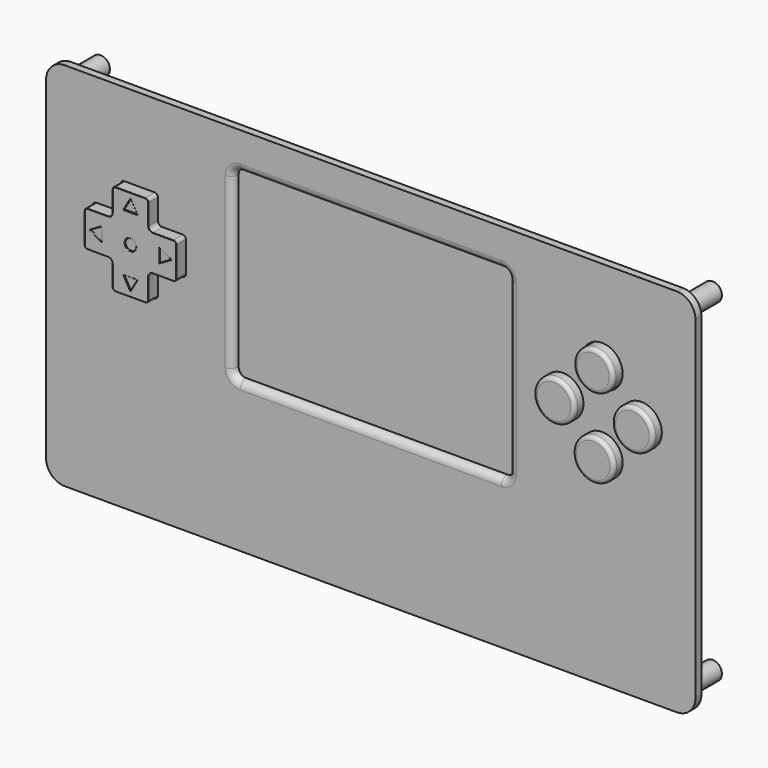
from build123d import *

# Parameters (mm, degrees)
F0_W           = 174
F0_H           = 99.3
F0_R           = 17.5
F0_W_2         = 74
F0_H_2         = 49.3
F0_R_2         = 5.5
F1_DEPTH       = 2
F2_R           = 1
F3_R           = 5
F4_R           = 6.5
F4_R_2         = 5.5
F5_DEPTH       = 5
F6_R           = 19.5
F6_R_2         = 17.5
F7_DEPTH       = 5
F8_R           = 1.99999
F9_R           = 2.5
F9_R_2         = 1
F10_DEPTH      = 10
F11_DEPTH      = 2
F13_DEPTH      = 3
F13_DEPTH_BACK = 3
F14_R          = 5.3
F15_DEPTH      = 3
F15_DEPTH_BACK = 2
F14_R_2        = 5.5
F16_R          = 1
F16_2_R        = 1
F16_3_R        = 1
F16_4_R        = 1
F17_R          = 1.5
F18_DEPTH      = 0.2
F19_R          = 0.09999


# Not quite as in the source:
# - a fillet or chamfer is up to 0.001 mm smaller than in the source, because OpenCascade refuses the exact size


with BuildPart() as f1:
    # F0 (on Front) → F1 (new body)
    with BuildSketch(Plane.XZ):
        with Locations((0, -15)):
            Rectangle(F0_W, F0_H)
        with Locations((-62, 0)):
            Circle(F0_R, mode=Mode.SUBTRACT)
        Rectangle(F0_W_2, F0_H_2, mode=Mode.SUBTRACT)
        with Locations((62, -10.5)):
            Circle(F0_R_2, mode=Mode.SUBTRACT)
        with Locations((51.5, 0)):
            Circle(F0_R_2, mode=Mode.SUBTRACT)
        with Locations((72.5, 0)):
            Circle(F0_R_2, mode=Mode.SUBTRACT)
        with Locations((62, 10.5)):
            Circle(F0_R_2, mode=Mode.SUBTRACT)
        with Locations((-62, 0)):
            Circle(F0_R)
        Polygon((-57, -5), (-57, -12.5), (-67, -12.5), (-67, -5), (-74.5, -5), (-74.5, 5), (-67, 5), (-67, 12.5), (-57, 12.5), (-57, 5), (-49.5, 5), (-49.5, -5), align=None, mode=Mode.SUBTRACT)
    extrude(amount=F1_DEPTH)

    # F2
    f2_edges = [f1.edges().sort_by_distance(p)[0] for p in [
        (-67, -1, 12.5),
        (-67, -1, 5),
        (-74.5, -1, 5),
        (-74.5, -1, -5),
        (-67, -1, -5),
        (-67, -1, -12.5),
        (-57, -1, -12.5),
        (-57, -1, -5),
        (-49.5, -1, -5),
        (-49.5, -1, 5),
        (-57, -1, 5),
        (-57, -1, 12.5),
    ]]
    fillet(f2_edges, radius=F2_R)

    # F3
    f3_edges = [f1.edges().sort_by_distance(p)[0] for p in [
        (87, -1, 34.65),
        (87, -1, -64.65),
        (-87, -1, 34.65),
        (-87, -1, -64.65),
    ]]
    fillet(f3_edges, radius=F3_R)

    # F4 (on face) → F5 (join)
    with BuildSketch(Plane(origin=(0, 0, 0), x_dir=(-1, 0, 0), z_dir=(0, 1, 0))):
        with Locations((-62, 10.5)):
            Circle(F4_R)
        with Locations((-62, 10.5)):
            Circle(F4_R_2, mode=Mode.SUBTRACT)
        with Locations((-72.5, 0)):
            Circle(F4_R)
        with Locations((-72.5, 0)):
            Circle(F4_R_2, mode=Mode.SUBTRACT)
        with Locations((-51.5, 0)):
            Circle(F4_R)
        with Locations((-51.5, 0)):
            Circle(F4_R_2, mode=Mode.SUBTRACT)
        with Locations((-62, -10.5)):
            Circle(F4_R)
        with Locations((-62, -10.5)):
            Circle(F4_R_2, mode=Mode.SUBTRACT)
    extrude(amount=F5_DEPTH)

    # F6 (on face) → F7 (join, through all)
    with BuildSketch(Plane.XZ):
        with Locations((-62, 0)):
            Circle(F6_R)
        with Locations((-62, 0)):
            Circle(F6_R_2, mode=Mode.SUBTRACT)
    extrude(amount=-F7_DEPTH)

    # F8 (radius 2 in the source; OpenCascade refuses exactly that, so slightly less here)
    f8_edges = [f1.edges().sort_by_distance(p)[0] for p in [
        (-37, -1, 24.65),
        (37, -1, 24.65),
        (37, -1, -24.65),
        (-37, -1, -24.65),
        (-37, -2, 0),
        (37, -2, 0),
        (0, -2, 24.65),
        (0, -2, -24.65),
    ]]
    fillet(f8_edges, radius=F8_R)

    # F9 (on face) → F10 (join)
    with BuildSketch(Plane.XZ):
        with Locations((82, 29.65)):
            Circle(F9_R)
        with Locations((82, 29.65)):
            Circle(F9_R_2, mode=Mode.SUBTRACT)
        with Locations((-82, 29.65)):
            Circle(F9_R)
        with Locations((-82, 29.65)):
            Circle(F9_R_2, mode=Mode.SUBTRACT)
        with Locations((-82, -59.65)):
            Circle(F9_R)
        with Locations((-82, -59.65)):
            Circle(F9_R_2, mode=Mode.SUBTRACT)
        with Locations((82, -59.65)):
            Circle(F9_R)
        with Locations((82, -59.65)):
            Circle(F9_R_2, mode=Mode.SUBTRACT)
    extrude(amount=-F10_DEPTH)


with BuildPart() as f11:
    # F0 (on Front) → F11 (new body)
    with BuildSketch(Plane.XZ):
        Rectangle(F0_W_2, F0_H_2)
    extrude(amount=-F11_DEPTH)


with BuildPart() as f13:
    # F12 (on face) → F13 (new body, two sides)
    with BuildSketch(Plane.XZ.offset(2)) as f13_sk:
        with BuildLine():
            ThreePointArc((-66.8, 6), (-67.1514718626, 5.1514718626), (-68, 4.8))
            Line((-68, 4.8), (-73.5, 4.8))
            ThreePointArc((-73.5, 4.8), (-74.0656854249, 4.5656854249), (-74.3, 4))
            Line((-74.3, 4), (-74.3, -4))
            ThreePointArc((-74.3, -4), (-74.0656854249, -4.5656854249), (-73.5, -4.8))
            Line((-73.5, -4.8), (-68, -4.8))
            ThreePointArc((-68, -4.8), (-67.1514718626, -5.1514718626), (-66.8, -6))
            Line((-66.8, -6), (-66.8, -11.5))
            ThreePointArc((-66.8, -11.5), (-66.5656854249, -12.0656854249), (-66, -12.3))
            Line((-66, -12.3), (-58, -12.3))
            ThreePointArc((-58, -12.3), (-57.4343145751, -12.0656854249), (-57.2, -11.5))
            Line((-57.2, -11.5), (-57.2, -6))
            ThreePointArc((-57.2, -6), (-56.8485281374, -5.1514718626), (-56, -4.8))
            Line((-56, -4.8), (-50.5, -4.8))
            ThreePointArc((-50.5, -4.8), (-49.9343145751, -4.5656854249), (-49.7, -4))
            Line((-49.7, -4), (-49.7, 4))
            ThreePointArc((-49.7, 4), (-49.9343145751, 4.5656854249), (-50.5, 4.8))
            Line((-50.5, 4.8), (-56, 4.8))
            ThreePointArc((-56, 4.8), (-56.8485281374, 5.1514718626), (-57.2, 6))
            Line((-57.2, 6), (-57.2, 11.5))
            ThreePointArc((-57.2, 11.5), (-57.4343145751, 12.0656854249), (-58, 12.3))
            Line((-58, 12.3), (-66, 12.3))
            ThreePointArc((-66, 12.3), (-66.5656854249, 12.0656854249), (-66.8, 11.5))
            Line((-66.8, 11.5), (-66.8, 6))
        make_face()
    extrude(amount=F13_DEPTH)
    extrude(f13_sk.sketch, amount=-F13_DEPTH_BACK)

    # F17 (on face) → F18 (cut)
    with BuildSketch(Plane.XZ.offset(5)):
        Polygon((-62, 10.8974880576), (-63.8597792122, 7.6762559712), (-60.1402207878, 7.6762559712), align=None)
        Polygon((-54.3237440288, 1.8597792122), (-54.3237440288, -1.8597792122), (-51.1025119424, 0), align=None)
        Polygon((-62, -10.8974880576), (-60.1402207878, -7.6762559712), (-63.8597792122, -7.6762559712), align=None)
        Polygon((-72.8974880576, 0), (-69.6762559712, -1.8597792122), (-69.6762559712, 1.8597792122), align=None)
        with Locations((-62, 0)):
            Circle(F17_R)
    extrude(amount=-F18_DEPTH, mode=Mode.SUBTRACT)

    # F19 (radius 0.1 in the source; OpenCascade refuses exactly that, so slightly less here)
    f19_edges = [f13.edges().sort_by_distance(p)[0] for p in [
        (-63.5, -4.8, 0),
        (-70.75, -5, -4.8),
        (-74.065685, -5, -4.565685),
        (-67.151472, -5, -5.151472),
        (-74.3, -5, 0),
        (-66.8, -5, -8.75),
        (-74.065685, -5, 4.565685),
        (-66.565685, -5, -12.065685),
        (-70.75, -5, 4.8),
        (-62, -5, -12.3),
        (-67.151472, -5, 5.151472),
        (-57.434315, -5, -12.065685),
        (-66.8, -5, 8.75),
        (-57.2, -5, -8.75),
        (-66.565685, -5, 12.065685),
        (-56.848528, -5, -5.151472),
        (-62, -5, 12.3),
        (-53.25, -5, -4.8),
        (-57.434315, -5, 12.065685),
        (-49.934315, -5, -4.565685),
        (-57.2, -5, 8.75),
        (-49.7, -5, 0),
        (-56.848528, -5, 5.151472),
        (-49.934315, -5, 4.565685),
        (-53.25, -5, 4.8),
        (-71.286872, -5, -0.92989),
        (-69.676256, -5, 0),
        (-71.286872, -5, 0.92989),
        (-62.92989, -5, -9.286872),
        (-61.07011, -5, -9.286872),
        (-62, -5, -7.676256),
        (-63.5, -5, 0),
        (-54.323744, -5, 0),
        (-52.713128, -5, -0.92989),
        (-52.713128, -5, 0.92989),
        (-62.92989, -5, 9.286872),
        (-62, -5, 7.676256),
        (-61.07011, -5, 9.286872),
        (-63.859779, -4.9, 7.676256),
        (-62, -4.9, 10.897488),
        (-62, -4.8, 7.676256),
        (-61.07011, -4.8, 9.286872),
        (-62.92989, -4.8, 9.286872),
        (-60.140221, -4.9, 7.676256),
        (-54.323744, -4.8, 0),
        (-52.713128, -4.8, -0.92989),
        (-52.713128, -4.8, 0.92989),
        (-54.323744, -4.9, -1.859779),
        (-51.102512, -4.9, 0),
        (-54.323744, -4.9, 1.859779),
        (-63.859779, -4.9, -7.676256),
        (-60.140221, -4.9, -7.676256),
        (-62, -4.9, -10.897488),
        (-62.92989, -4.8, -9.286872),
        (-61.07011, -4.8, -9.286872),
        (-62, -4.8, -7.676256),
        (-71.286872, -4.8, -0.92989),
        (-71.286872, -4.8, 0.92989),
        (-69.676256, -4.9, 1.859779),
        (-72.897488, -4.9, 0),
        (-69.676256, -4.9, -1.859779),
        (-69.676256, -4.8, 0),
    ]]
    fillet(f19_edges, radius=F19_R)


with BuildPart() as f15:
    # F14 (on face) → F15 (new body, two sides)
    with BuildSketch(Plane.XZ.offset(2)) as f15_sk:
        with Locations((62, 10.5)):
            Circle(F14_R)
    extrude(amount=F15_DEPTH)
    extrude(f15_sk.sketch, amount=-F15_DEPTH_BACK)

    # F16
    f16_edges = [f15.edges().sort_by_distance(p)[0] for p in [
        (56.7, -5, 10.5),
    ]]
    fillet(f16_edges, radius=F16_R)


with BuildPart() as f15b:
    # F14 (on face) → F15, piece 2 (new body, two sides)
    with BuildSketch(Plane.XZ.offset(2)) as f15_2_sk:
        with Locations((51.5, 0)):
            Circle(F14_R_2)
    extrude(amount=F15_DEPTH)
    extrude(f15_2_sk.sketch, amount=-F15_DEPTH_BACK)

    # F16#2
    f16_2_edges = [f15b.edges().sort_by_distance(p)[0] for p in [
        (46, -5, 0),
    ]]
    fillet(f16_2_edges, radius=F16_2_R)


with BuildPart() as f15c:
    # F14 (on face) → F15, piece 3 (new body, two sides)
    with BuildSketch(Plane.XZ.offset(2)) as f15_3_sk:
        with Locations((72.5, 0)):
            Circle(F14_R_2)
    extrude(amount=F15_DEPTH)
    extrude(f15_3_sk.sketch, amount=-F15_DEPTH_BACK)

    # F16#3
    f16_3_edges = [f15c.edges().sort_by_distance(p)[0] for p in [
        (67, -5, 0),
    ]]
    fillet(f16_3_edges, radius=F16_3_R)


with BuildPart() as f15d:
    # F14 (on face) → F15, piece 4 (new body, two sides)
    with BuildSketch(Plane.XZ.offset(2)) as f15_4_sk:
        with Locations((62, -10.5)):
            Circle(F14_R_2)
    extrude(amount=F15_DEPTH)
    extrude(f15_4_sk.sketch, amount=-F15_DEPTH_BACK)

    # F16#4
    f16_4_edges = [f15d.edges().sort_by_distance(p)[0] for p in [
        (56.5, -5, -10.5),
    ]]
    fillet(f16_4_edges, radius=F16_4_R)


solid = Compound([f1.part, f11.part, f13.part, f15.part, f15b.part, f15c.part, f15d.part])
